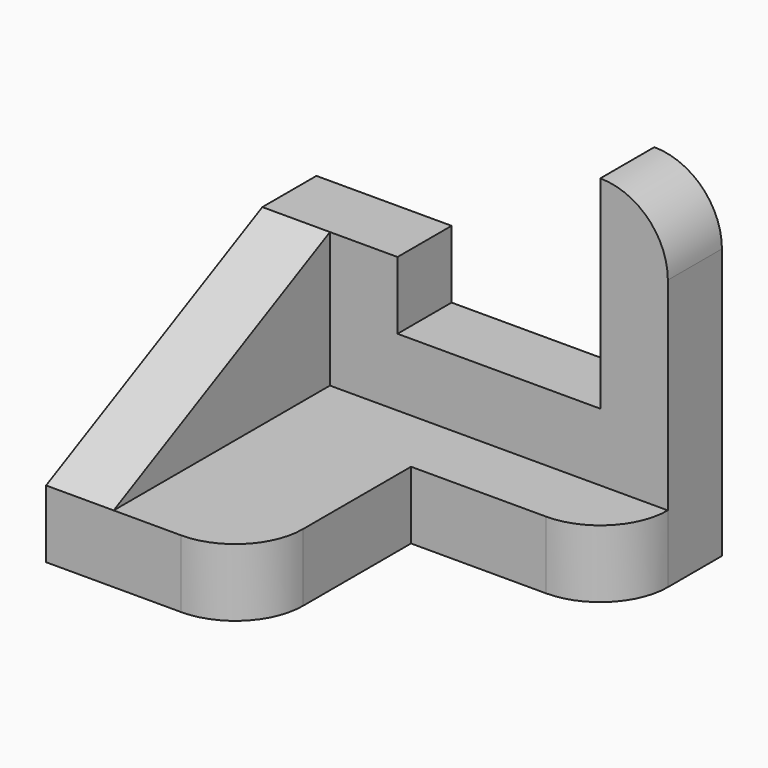
from build123d import *

# Parameters (mm, degrees)
F1_DEPTH = 10
F0_W     = 30
F0_H     = 10
F2_DEPTH = 20
F3_DEPTH = 30
F0_W_2   = 10
F4_DEPTH = 50
F0_H_2   = 40
F5_DEPTH = 30
F6_R     = 9.99999
F7_SIZE2 = 20
F7_SIZE  = 40


# Not quite as in the source:
# - a fillet or chamfer is up to 0.001 mm smaller than in the source, because OpenCascade refuses the exact size


with BuildPart() as f1:
    # F0 (on Top) → F1 (new body)
    with BuildSketch(Plane.XY):
        with BuildLine():
            ThreePointArc((11.2901248038, 30), (18.3611926156, 32.9289321881), (21.2901248038, 40))
            Line((21.2901248038, 40), (11.2901248038, 40))
            Line((11.2901248038, 40), (-18.7098751962, 40))
            Line((-18.7098751962, 40), (-28.7098751962, 40))
            Line((-28.7098751962, 40), (-28.7098751962, 0))
            Line((-28.7098751962, 0), (-18.7098751962, 0))
            ThreePointArc((-18.7098751962, 0), (-11.6388073844, 2.9289321881), (-8.7098751962, 10))
            Line((-8.7098751962, 10), (-8.7098751962, 30))
            Line((-8.7098751962, 30), (11.2901248038, 30))
        make_face()
    extrude(amount=F1_DEPTH)

    # F0 (on Top) → F2 (join)
    with BuildSketch(Plane.XY):
        with Locations((-3.7098751962, 45)):
            Rectangle(F0_W, F0_H)
    extrude(amount=F2_DEPTH)

    # F0 (on Top) → F3 (join)
    with BuildSketch(Plane.XY):
        Polygon((-28.7098751962, 40), (-18.7098751962, 40), (-18.7098751962, 50), (-38.7098751962, 50), (-38.7098751962, 40), align=None)
    extrude(amount=F3_DEPTH)

    # F0 (on Top) → F4 (join)
    with BuildSketch(Plane.XY):
        with Locations((16.2901248038, 45)):
            Rectangle(F0_W_2, F0_H)
    extrude(amount=F4_DEPTH)

    # F0 (on Top) → F5 (join)
    with BuildSketch(Plane.XY):
        with Locations((-33.7098751962, 20)):
            Rectangle(F0_W_2, F0_H_2)
    extrude(amount=F5_DEPTH)

    # F6 (radius 10 in the source; OpenCascade refuses exactly that, so slightly less here)
    f6_edges = [f1.edges().sort_by_distance(p)[0] for p in [
        (21.290125, 45, 50),
    ]]
    fillet(f6_edges, radius=F6_R)

    # F7
    f7_edges = [f1.edges().sort_by_distance(p)[0] for p in [
        (-33.709875, 0, 30),
    ]]
    f7_side = f1.faces().sort_by_distance((-32.043209, 28.333333, 30))[0]
    chamfer(f7_edges, length=F7_SIZE, length2=F7_SIZE2, reference=f7_side)


solid = f1.part
